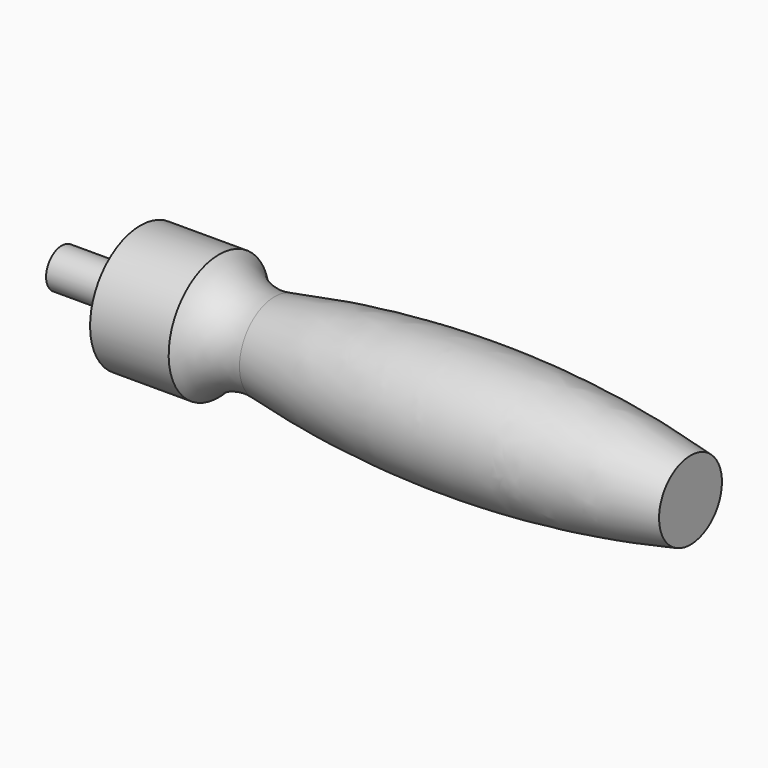
from build123d import *

# Parameters (mm, degrees)
F0_W = 10
F0_H = 2.5


# Not quite as in the source:
# - a fillet or chamfer that OpenCascade refuses, or shapes differently, is made with other operations: its cross-section is extruded or revolved along the edge and cut away or added


with BuildPart() as f1:
    # F0 (on Front) → F1 (revolve)
    with BuildSketch(Plane.XZ):
        with Locations((-5, 1.25)):
            Rectangle(F0_W, F0_H)
        Polygon((0, 8), (0, 2.5), (0, 0), (10, 0), (10, 4), (10, 8), align=None)
        with BuildLine():
            Line((10, 4), (10, 0))
            Line((10, 0), (70, 0))
            Line((70, 0), (70, 5))
            ThreePointArc((70, 5), (39.9419698495, 7.9818090321), (10, 4))
        make_face()
    revolve(axis=Axis((40, 0, 0), (1, 0, 0)))

    # F2: fillet of radius 7.5 on 1 edges, made by hand

    # F2_s1 → F2_t2 (revolve)
    with BuildSketch(Plane.XZ):
        with BuildLine():
            ThreePointArc((17.0739020896, 5.582469697), (13.2142793321, 5.8470695986), (10, 8))
            Line((10, 8), (10, 4))
            ThreePointArc((10, 4), (13.5260036045, 4.8401717227), (17.0739020896, 5.582469697))
        make_face()
    revolve(axis=Axis((10, 0, 0), (1, 0, 0)))


solid = f1.part
